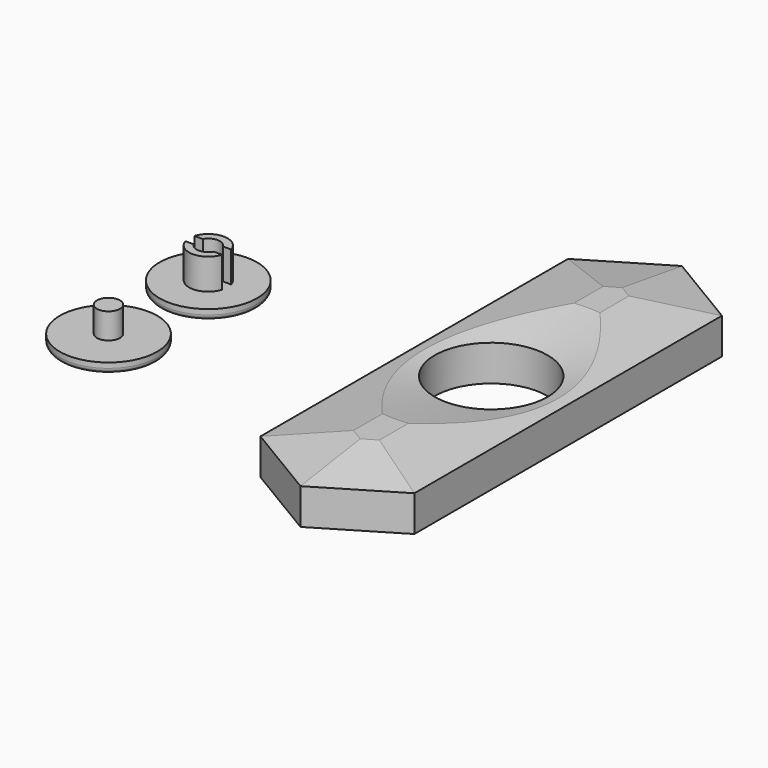
from build123d import *

# Parameters (mm, degrees)
F0_R       = 11
F1_DEPTH   = 3.5
F3_DEPTH   = 8
F2_R       = 9.5
F4_DEPTH   = 2
F5_R       = 1
F6_R       = 9.5
F6_R_2     = 2.25
F7_DEPTH   = 2
F8_DEPTH   = 7
F9_R       = 1
F1_FACE_R  = 11
F1_FACE1_R = 11
F10_DEPTH  = 2.2
F10_TAPER  = 80


# Not quite as in the source:
# - a feature names something its author has since deleted; it is built from what else it names


with BuildPart() as f1:
    # F0 (on Top) → F1 (new body, symmetric)
    with BuildSketch(Plane.XY):
        Polygon((0, -46.4706834555), (15, -37.4706834555), (15, 37.4706834555), (0, 46.4706834555), (-15, 37.4706834555), (-15, -37.4706834555), align=None)
        Circle(F0_R, mode=Mode.SUBTRACT)
    extrude(amount=F1_DEPTH, both=True)

    # F1_face (on face) + F1_face1 (on face) → F10 (join, symmetric)
    with BuildSketch(Plane.XY.offset(3.5)):
        Polygon((-15, -37.4706834555), (0, -46.4706834555), (15, -37.4706834555), (15, 37.4706834555), (0, 46.4706834555), (-15, 37.4706834555), align=None)
        Circle(F1_FACE_R, mode=Mode.SUBTRACT)
    with BuildSketch(Plane(origin=(0, 0, -3.5), x_dir=(1, 0, 0), z_dir=(0, 0, -1))):
        Polygon((0, 46.4706834555), (-15, 37.4706834555), (-15, -37.4706834555), (0, -46.4706834555), (15, -37.4706834555), (15, 37.4706834555), align=None)
        Circle(F1_FACE1_R, mode=Mode.SUBTRACT)
    extrude(amount=F10_DEPTH, both=True, taper=F10_TAPER, dir=(0, 0, 1))


with BuildPart() as f3:
    # F2 (on Top) → F3 (new body)
    with BuildSketch(Plane.XY):
        with BuildLine():
            Line((-53.1808868797, 1.1), (-51.5586271683, 1.1))
            ThreePointArc((-51.5586271683, 1.1), (-55.1436655223, 3.75), (-58.7287038764, 1.1))
            Line((-58.7287038764, 1.1), (-57.106444165, 1.1))
            ThreePointArc((-57.106444165, 1.1), (-55.1436655223, 2.25), (-53.1808868797, 1.1))
        make_face()
    extrude(amount=F3_DEPTH)



with BuildPart() as f3b:
    # F2 (on Top) → F3, piece 2 (new body)
    with BuildSketch(Plane.XY):
        with BuildLine():
            ThreePointArc((-58.7287038764, -1.1), (-55.1436655223, -3.75), (-51.5586271683, -1.1))
            Line((-51.5586271683, -1.1), (-53.1808868797, -1.1))
            ThreePointArc((-53.1808868797, -1.1), (-55.1436655223, -2.25), (-57.106444165, -1.1))
            Line((-57.106444165, -1.1), (-58.7287038764, -1.1))
        make_face()
    extrude(amount=F3_DEPTH)


with BuildPart() as f3_1:
    add(f3.part)

    add(f3b.part)  # F4 merges F3b
    # F2 (on Top) → F4 (join)
    with BuildSketch(Plane.XY):
        with Locations((-55.1436655223, 0)):
            Circle(F2_R)
        with BuildLine():
            ThreePointArc((-51.5586271683, 1.1), (-51.4351352321, 0.556150237), (-51.3936655223, 0))
            ThreePointArc((-51.3936655223, 0), (-51.4351352321, -0.556150237), (-51.5586271683, -1.1))
            ThreePointArc((-51.5586271683, -1.1), (-55.1436655223, -3.75), (-58.7287038764, -1.1))
            ThreePointArc((-58.7287038764, -1.1), (-58.8936655223, 0), (-58.7287038764, 1.1))
            ThreePointArc((-58.7287038764, 1.1), (-55.1436655223, 3.75), (-51.5586271683, 1.1))
        make_face(mode=Mode.SUBTRACT)
        with BuildLine():
            ThreePointArc((-52.8936655223, 0), (-52.9666547339, 0.5684399942), (-53.1808868797, 1.1))
            Line((-53.1808868797, 1.1), (-57.106444165, 1.1))
            ThreePointArc((-57.106444165, 1.1), (-57.3936655223, 0), (-57.106444165, -1.1))
            Line((-57.106444165, -1.1), (-53.1808868797, -1.1))
            ThreePointArc((-53.1808868797, -1.1), (-52.9666547339, -0.5684399942), (-52.8936655223, 0))
        make_face()
        with BuildLine():
            Line((-51.5586271683, -1.1), (-51.5586271683, 1.1))
            Line((-51.5586271683, 1.1), (-53.1808868797, 1.1))
            ThreePointArc((-53.1808868797, 1.1), (-52.9666547339, 0.5684399942), (-52.8936655223, 0))
            ThreePointArc((-52.8936655223, 0), (-52.9666547339, -0.5684399942), (-53.1808868797, -1.1))
            Line((-53.1808868797, -1.1), (-51.5586271683, -1.1))
        make_face()
        with BuildLine():
            Line((-57.106444165, 1.1), (-53.1808868797, 1.1))
            ThreePointArc((-53.1808868797, 1.1), (-55.1436655223, 2.25), (-57.106444165, 1.1))
        make_face()
        with BuildLine():
            ThreePointArc((-57.106444165, -1.1), (-55.1436655223, -2.25), (-53.1808868797, -1.1))
            Line((-53.1808868797, -1.1), (-57.106444165, -1.1))
        make_face()
        with BuildLine():
            Line((-58.7287038764, -1.1), (-58.7287038764, 1.1))
            ThreePointArc((-58.7287038764, 1.1), (-58.8936655223, 0), (-58.7287038764, -1.1))
        make_face()
        with BuildLine():
            Line((-57.106444165, 1.1), (-58.7287038764, 1.1))
            Line((-58.7287038764, 1.1), (-58.7287038764, -1.1))
            Line((-58.7287038764, -1.1), (-57.106444165, -1.1))
            ThreePointArc((-57.106444165, -1.1), (-57.3936655223, 0), (-57.106444165, 1.1))
        make_face()
        with BuildLine():
            ThreePointArc((-51.5586271683, -1.1), (-51.4351352321, -0.556150237), (-51.3936655223, 0))
            ThreePointArc((-51.3936655223, 0), (-51.4351352321, 0.556150237), (-51.5586271683, 1.1))
            Line((-51.5586271683, 1.1), (-51.5586271683, -1.1))
        make_face()
    extrude(amount=F4_DEPTH)

    # F5
    f5_edges = [f3_1.edges().sort_by_distance(p)[0] for p in [
        (-64.643666, 0, 0),
    ]]
    fillet(f5_edges, radius=F5_R)


with BuildPart() as f7:
    # F6 (on Top) → F7 (new body)
    with BuildSketch(Plane.XY):
        with Locations((-56.0084953904, -23.2402067631)):
            Circle(F6_R)
        with Locations((-56.0084953904, -23.2402067631)):
            Circle(F6_R_2, mode=Mode.SUBTRACT)
    extrude(amount=F7_DEPTH)

    # F6 (on Top) → F8 (join)
    with BuildSketch(Plane.XY):
        with Locations((-56.0084953904, -23.2402067631)):
            Circle(F6_R_2)
    extrude(amount=F8_DEPTH)

    # F9
    f9_edges = [f7.edges().sort_by_distance(p)[0] for p in [
        (-65.508495, -23.240207, 0),
    ]]
    fillet(f9_edges, radius=F9_R)


solid = Compound([f1.part, f3_1.part, f7.part])
